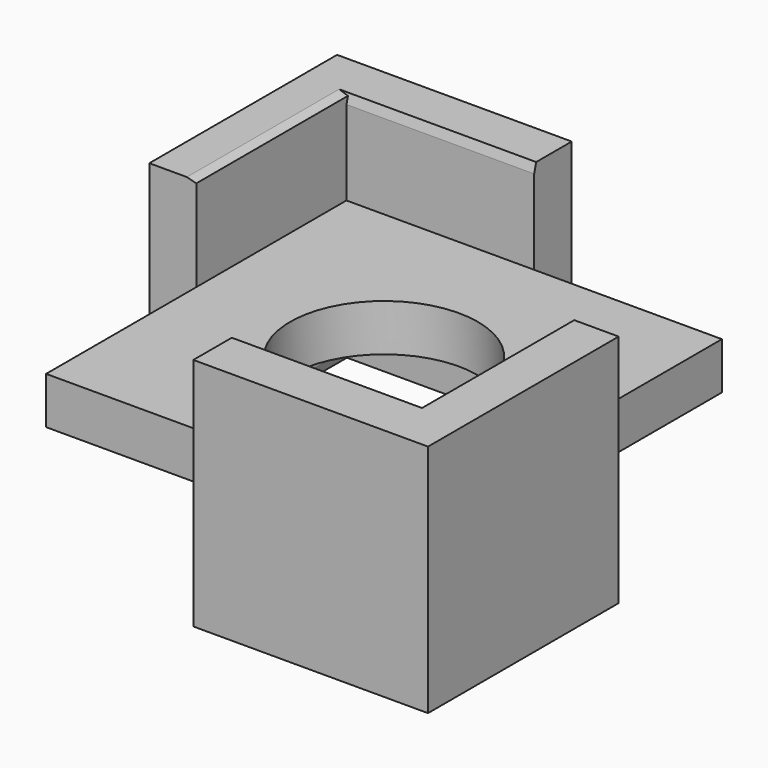
from build123d import *

# Parameters (mm, degrees)
F0_W          = 50.8
F0_H          = 50.8
F3_DEPTH      = 3.175
F4_DEPTH      = 15.875
F5_DEPTH      = 15.875
F6_T1_DEPTH   = 28.6978363942
F6_T3_DEPTH   = 28.6978363942
F6_T5_DEPTH   = 28.6978363942
F6_T7_DEPTH   = 28.6978363942
F6_T13_DEPTH  = 31.9956727883
F6_T17_DEPTH  = 31.9956727883
F6_T24_DEPTH  = 31.9956727883
F6_T28_DEPTH  = 31.9956727883
F6_T35_DEPTH  = 31.9956727883
F6_T39_DEPTH  = 31.9956727883
F6_T46_DEPTH  = 31.9956727883
F6_T50_DEPTH  = 31.9956727883
F7_R          = 12.7
F8_DEPTH      = 15.876
F8_DEPTH_BACK = 15.876


# Not quite as in the source:
# - a fillet or chamfer that OpenCascade refuses, or shapes differently, is made with other operations: its cross-section is extruded or revolved along the edge and cut away or added


with BuildPart() as f3:
    # F0 (on Top) → F3 (new body, symmetric)
    with BuildSketch(Plane.XY):
        with Locations((-25.4, 25.4)):
            Rectangle(F0_W, F0_H)
    extrude(amount=F3_DEPTH, both=True)

    # F1 (on Top) → F4 (join, symmetric)
    with BuildSketch(Plane.XY):
        Polygon((0, 25.4), (0, 0), (-25.4, 0), (-25.4, -6.8448194891), (6.35, -6.8448194891), (6.35, 25.4), align=None)
    extrude(amount=F4_DEPTH, both=True)

    # F2 (on Top) → F5 (join, symmetric)
    with BuildSketch(Plane.XY):
        Polygon((-50.8, 50.8), (-25.4, 50.8), (-25.4, 57.15), (-57.15, 57.15), (-57.15, 25.4), (-50.8, 25.4), align=None)
    extrude(amount=F5_DEPTH, both=True)

    # F6: chamfer of 1.27 x 0.3402954744 on 8 edges, made by hand

    # F6_s2 → F6_t1 (cut)
    with BuildSketch(Plane.YZ.offset(-28.6978363942)):
        Polygon((0, 14.605), (-0.3402954744, 15.875), (0, 15.875), align=None)
        Polygon((-1.27, -15.875), (0, -15.5347045256), (0, -15.875), align=None)
    extrude(amount=F6_T1_DEPTH, mode=Mode.SUBTRACT)

    # F6_s4 → F6_t3 (cut)
    with BuildSketch(Plane.XZ.offset(-28.6978363942)):
        Polygon((0, 14.605), (0.3402954744, 15.875), (0, 15.875), align=None)
        Polygon((1.27, -15.875), (0, -15.5347045256), (0, -15.875), align=None)
    extrude(amount=F6_T3_DEPTH, mode=Mode.SUBTRACT)

    # F6_s6 → F6_t5 (cut)
    with BuildSketch(Plane.YZ.offset(-50.8)):
        Polygon((50.8, 14.605), (51.1402954744, 15.875), (50.8, 15.875), align=None)
        Polygon((50.8, -15.5347045256), (52.07, -15.875), (50.8, -15.875), align=None)
    extrude(amount=F6_T5_DEPTH, mode=Mode.SUBTRACT)

    # F6_s8 → F6_t7 (cut)
    with BuildSketch(Plane.XZ.offset(-50.8)):
        Polygon((-50.8, 15.5347045256), (-52.07, 15.875), (-50.8, 15.875), align=None)
        Polygon((-50.8, -14.605), (-51.1402954744, -15.875), (-50.8, -15.875), align=None)
    extrude(amount=F6_T7_DEPTH, mode=Mode.SUBTRACT)


with BuildPart() as f6_tool11:
    # F6_s12 → F6_t13 (new body)
    with BuildSketch(Plane.YZ.offset(3.2978363942)):
        Polygon((0, 14.605), (-0.3402954744, 15.875), (0, 15.875), align=None)
    extrude(amount=-F6_T13_DEPTH)

    split(bisect_by=Plane.YZ, keep=Keep.TOP)


with BuildPart() as f6_tool15:
    # F6_s16 → F6_t17 (new body)
    with BuildSketch(Plane.XZ.offset(-28.6978363942)):
        Polygon((0, 14.605), (0.3402954744, 15.875), (0, 15.875), align=None)
    extrude(amount=F6_T17_DEPTH)

    split(bisect_by=Plane.XZ, keep=Keep.TOP)


with BuildPart() as f6_tool11_1:
    add(f6_tool11.part)

    # F6_t19: intersect F6_tool15
    add(f6_tool15.part, mode=Mode.INTERSECT)


with BuildPart() as f3_1:
    add(f3.part)

    # F6_t9: cut F6_tool11
    add(f6_tool11_1.part, mode=Mode.SUBTRACT)


with BuildPart() as f6_tool22:
    # F6_s23 → F6_t24 (new body)
    with BuildSketch(Plane.YZ.offset(-54.0978363942)):
        Polygon((50.8, 14.605), (51.1402954744, 15.875), (50.8, 15.875), align=None)
    extrude(amount=F6_T24_DEPTH)

    split(bisect_by=Plane.YZ.offset(-50.8), keep=Keep.BOTTOM)


with BuildPart() as f6_tool26:
    # F6_s27 → F6_t28 (new body)
    with BuildSketch(Plane.XZ.offset(-22.1021636058)):
        Polygon((-50.8, 15.5347045256), (-52.07, 15.875), (-50.8, 15.875), align=None)
    extrude(amount=-F6_T28_DEPTH)

    split(bisect_by=Plane.XZ.offset(-50.8), keep=Keep.BOTTOM)


with BuildPart() as f6_tool22_1:
    add(f6_tool22.part)

    # F6_t30: intersect F6_tool26
    add(f6_tool26.part, mode=Mode.INTERSECT)


with BuildPart() as f3_2:
    add(f3_1.part)

    # F6_t20: cut F6_tool22
    add(f6_tool22_1.part, mode=Mode.SUBTRACT)


with BuildPart() as f6_tool33:
    # F6_s34 → F6_t35 (new body)
    with BuildSketch(Plane.XZ.offset(-28.6978363942)):
        Polygon((1.27, -15.875), (0, -15.5347045256), (0, -15.875), align=None)
    extrude(amount=F6_T35_DEPTH)

    split(bisect_by=Plane.XZ, keep=Keep.TOP)


with BuildPart() as f6_tool37:
    # F6_s38 → F6_t39 (new body)
    with BuildSketch(Plane.YZ.offset(3.2978363942)):
        Polygon((-1.27, -15.875), (0, -15.5347045256), (0, -15.875), align=None)
    extrude(amount=-F6_T39_DEPTH)

    split(bisect_by=Plane.YZ, keep=Keep.TOP)


with BuildPart() as f6_tool33_1:
    add(f6_tool33.part)

    # F6_t41: intersect F6_tool37
    add(f6_tool37.part, mode=Mode.INTERSECT)


with BuildPart() as f3_3:
    add(f3_2.part)

    # F6_t31: cut F6_tool33
    add(f6_tool33_1.part, mode=Mode.SUBTRACT)


with BuildPart() as f6_tool44:
    # F6_s45 → F6_t46 (new body)
    with BuildSketch(Plane.YZ.offset(-54.0978363942)):
        Polygon((50.8, -15.5347045256), (52.07, -15.875), (50.8, -15.875), align=None)
    extrude(amount=F6_T46_DEPTH)

    split(bisect_by=Plane.YZ.offset(-50.8), keep=Keep.BOTTOM)


with BuildPart() as f6_tool48:
    # F6_s49 → F6_t50 (new body)
    with BuildSketch(Plane.XZ.offset(-22.1021636058)):
        Polygon((-50.8, -14.605), (-51.1402954744, -15.875), (-50.8, -15.875), align=None)
    extrude(amount=-F6_T50_DEPTH)

    split(bisect_by=Plane.XZ.offset(-50.8), keep=Keep.BOTTOM)


with BuildPart() as f6_tool44_1:
    add(f6_tool44.part)

    # F6_t52: intersect F6_tool48
    add(f6_tool48.part, mode=Mode.INTERSECT)


with BuildPart() as f3_4:
    add(f3_3.part)

    # F6_t42: cut F6_tool44
    add(f6_tool44_1.part, mode=Mode.SUBTRACT)

    # F7 (on Top) → F8 (cut, two sides)
    with BuildSketch(Plane.XY) as f8_sk:
        with Locations((-25.4, 25.4)):
            Circle(F7_R)
    extrude(amount=-F8_DEPTH, mode=Mode.SUBTRACT)
    extrude(f8_sk.sketch, amount=F8_DEPTH_BACK, mode=Mode.SUBTRACT)


solid = f3_4.part
